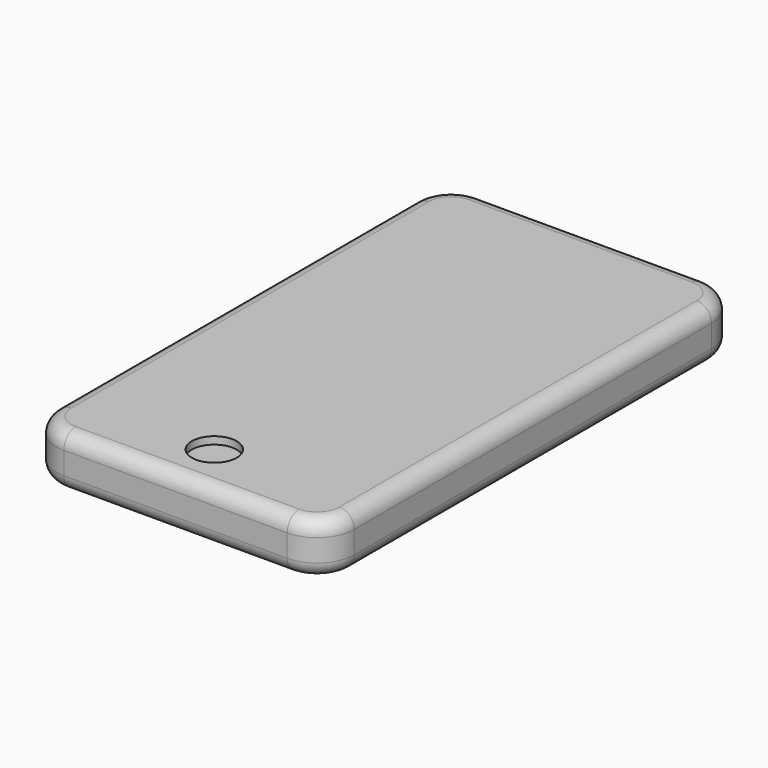
from build123d import *

# Parameters (mm, degrees)
F0_W         = 40
F0_H         = 70
F1_DEPTH     = 7
F2_R         = 5
F3_R         = 2
F4_DEPTH     = 3
F6_T1_DEPTH  = 60
F6_T3_DEPTH  = 30
F6_T6_ANGLE  = 90
F6_T8_ANGLE  = 90
F6_T10_ANGLE = 90
F6_T12_ANGLE = 90
F6_T14_ANGLE = 90
F6_T16_ANGLE = 90
F6_T18_ANGLE = 90
F6_T20_ANGLE = 90
F7_R         = 3.0179077215
F8_DEPTH     = 1


# Not quite as in the source:
# - a fillet or chamfer that OpenCascade refuses, or shapes differently, is made with other operations: its cross-section is extruded or revolved along the edge and cut away or added
# - a feature of the source that left no trace in its solid (it failed there, or was rolled back) is left out


with BuildPart() as f1:
    # F0 (on Top) → F1 (new body)
    with BuildSketch(Plane.XY):
        with Locations((20, 35)):
            Rectangle(F0_W, F0_H)
    extrude(amount=F1_DEPTH)

    # F2
    f2_edges = [f1.edges().sort_by_distance(p)[0] for p in [
        (40, 0, 3.5),
        (40, 70, 3.5),
        (0, 70, 3.5),
        (0, 0, 3.5),
    ]]
    fillet(f2_edges, radius=F2_R)

    # F3 (on face) → F4 (cut)
    with BuildSketch(Plane(origin=(0, 70, 0), x_dir=(-1, 0, 0), z_dir=(0, 1, 0))):
        with Locations((-31.323697418, 3.5)):
            Circle(F3_R)
    extrude(amount=-F4_DEPTH, mode=Mode.SUBTRACT)

    # F6: fillet of radius 2 on 16 edges, made by hand

    # F6_s2 → F6_t1 (cut)
    with BuildSketch(Plane.XZ.offset(-65)):
        with BuildLine():
            ThreePointArc((2, 7), (0.5857864376, 6.4142135624), (0, 5))
            Line((0, 5), (0, 7))
            Line((0, 7), (2, 7))
        make_face()
        with BuildLine():
            ThreePointArc((38, 0), (39.4142135624, 0.5857864376), (40, 2))
            Line((40, 2), (40, 0))
            Line((40, 0), (38, 0))
        make_face()
        with BuildLine():
            ThreePointArc((2, 0), (0.5857864376, 0.5857864376), (0, 2))
            Line((0, 2), (0, 0))
            Line((0, 0), (2, 0))
        make_face()
        with BuildLine():
            ThreePointArc((38, 7), (39.4142135624, 6.4142135624), (40, 5))
            Line((40, 5), (40, 7))
            Line((40, 7), (38, 7))
        make_face()
    extrude(amount=F6_T1_DEPTH, mode=Mode.SUBTRACT)

    # F6_s4 → F6_t3 (cut)
    with BuildSketch(Plane.YZ.offset(5)):
        with BuildLine():
            ThreePointArc((70, 2), (69.4142135624, 0.5857864376), (68, 0))
            Line((68, 0), (70, 0))
            Line((70, 0), (70, 2))
        make_face()
        with BuildLine():
            ThreePointArc((70, 5), (69.4142135624, 6.4142135624), (68, 7))
            Line((68, 7), (70, 7))
            Line((70, 7), (70, 5))
        make_face()
        with BuildLine():
            ThreePointArc((2, 0), (0.5857864376, 0.5857864376), (0, 2))
            Line((0, 2), (0, 0))
            Line((0, 0), (2, 0))
        make_face()
        with BuildLine():
            ThreePointArc((2, 7), (0.5857864376, 6.4142135624), (0, 5))
            Line((0, 5), (0, 7))
            Line((0, 7), (2, 7))
        make_face()
    extrude(amount=F6_T3_DEPTH, mode=Mode.SUBTRACT)

    # F6_s5 → F6_t6 (revolve, cut)
    with BuildSketch(Plane.YZ.offset(35)):
        with BuildLine():
            ThreePointArc((68, 0), (69.4142135624, 0.5857864376), (70, 2))
            Line((70, 2), (70, 0))
            Line((70, 0), (68, 0))
        make_face()
    revolve(axis=Axis((35, 65, 0), (0, 0, -1)), revolution_arc=F6_T6_ANGLE, mode=Mode.SUBTRACT)

    # F6_s7 → F6_t8 (revolve, cut)
    with BuildSketch(Plane.YZ.offset(5)):
        with BuildLine():
            ThreePointArc((68, 0), (69.4142135624, 0.5857864376), (70, 2))
            Line((70, 2), (70, 0))
            Line((70, 0), (68, 0))
        make_face()
    revolve(axis=Axis((5, 65, 0), (0, 0, 1)), revolution_arc=F6_T8_ANGLE, mode=Mode.SUBTRACT)

    # F6_s9 → F6_t10 (revolve, cut)
    with BuildSketch(Plane.YZ.offset(35)):
        with BuildLine():
            ThreePointArc((2, 0), (0.5857864376, 0.5857864376), (0, 2))
            Line((0, 2), (0, 0))
            Line((0, 0), (2, 0))
        make_face()
    revolve(axis=Axis((35, 5, 0), (0, 0, 1)), revolution_arc=F6_T10_ANGLE, mode=Mode.SUBTRACT)

    # F6_s11 → F6_t12 (revolve, cut)
    with BuildSketch(Plane.XZ.offset(-5)):
        with BuildLine():
            ThreePointArc((2, 0), (0.5857864376, 0.5857864376), (0, 2))
            Line((0, 2), (0, 0))
            Line((0, 0), (2, 0))
        make_face()
    revolve(axis=Axis((5, 5, 0), (0, 0, 1)), revolution_arc=F6_T12_ANGLE, mode=Mode.SUBTRACT)

    # F6_s13 → F6_t14 (revolve, cut)
    with BuildSketch(Plane.YZ.offset(35)):
        with BuildLine():
            ThreePointArc((70, 5), (69.4142135624, 6.4142135624), (68, 7))
            Line((68, 7), (70, 7))
            Line((70, 7), (70, 5))
        make_face()
    revolve(axis=Axis((35, 65, 7), (0, 0, -1)), revolution_arc=F6_T14_ANGLE, mode=Mode.SUBTRACT)

    # F6_s15 → F6_t16 (revolve, cut)
    with BuildSketch(Plane.YZ.offset(5)):
        with BuildLine():
            ThreePointArc((70, 5), (69.4142135624, 6.4142135624), (68, 7))
            Line((68, 7), (70, 7))
            Line((70, 7), (70, 5))
        make_face()
    revolve(axis=Axis((5, 65, 7), (0, 0, 1)), revolution_arc=F6_T16_ANGLE, mode=Mode.SUBTRACT)

    # F6_s17 → F6_t18 (revolve, cut)
    with BuildSketch(Plane.YZ.offset(35)):
        with BuildLine():
            ThreePointArc((2, 7), (0.5857864376, 6.4142135624), (0, 5))
            Line((0, 5), (0, 7))
            Line((0, 7), (2, 7))
        make_face()
    revolve(axis=Axis((35, 5, 7), (0, 0, 1)), revolution_arc=F6_T18_ANGLE, mode=Mode.SUBTRACT)

    # F6_s19 → F6_t20 (revolve, cut)
    with BuildSketch(Plane.XZ.offset(-5)):
        with BuildLine():
            ThreePointArc((2, 7), (0.5857864376, 6.4142135624), (0, 5))
            Line((0, 5), (0, 7))
            Line((0, 7), (2, 7))
        make_face()
    revolve(axis=Axis((5, 5, 7), (0, 0, 1)), revolution_arc=F6_T20_ANGLE, mode=Mode.SUBTRACT)

    # F7 (on face) → F8 (cut)
    with BuildSketch(Plane.XY.offset(7)):
        with Locations((19.5853062672, 7.0179077215)):
            Circle(F7_R)
    extrude(amount=-F8_DEPTH, mode=Mode.SUBTRACT)


solid = f1.part
